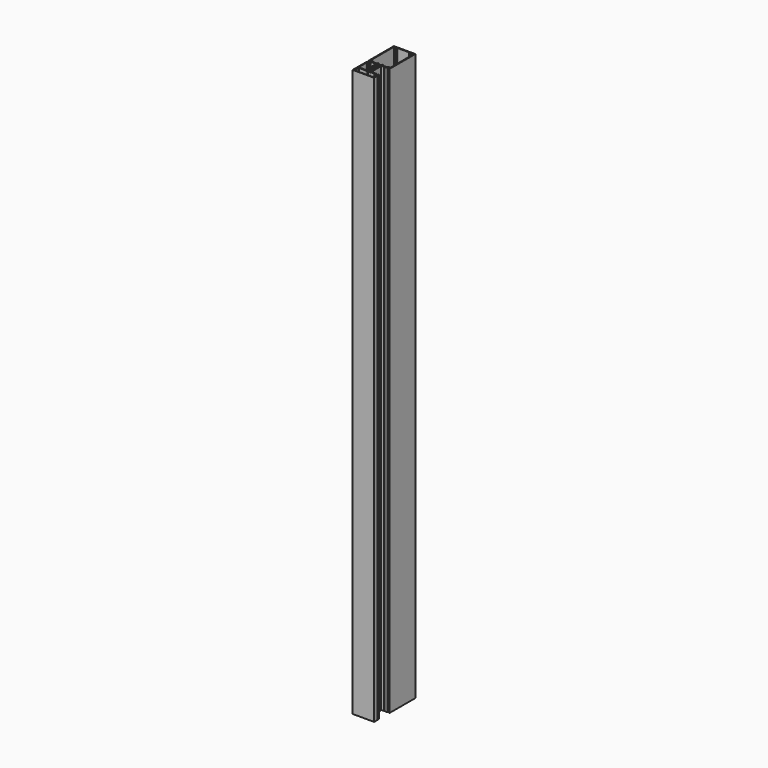
from build123d import *

# Parameters (mm, degrees)
F1_DEPTH = 838.2
F2_DEPTH = 838.2
F3_DEPTH = 838.2


# Not quite as in the source:
# - ends of sketch curves that miss each other by under 0.0002 mm in the source are joined


with BuildPart() as f1:
    # F0 (on Top) → F1 (new body, symmetric)
    with BuildSketch(Plane.XY):
        with BuildLine():
            Line((-36.0498644, -21.2344), (-36.0498644, -50.8))
            Line((-36.0498644, -50.8), (-35.0338644, -50.8))
            Line((-35.0338644, -50.8), (-34.6528644, -51.181))
            Line((-34.6528644, -51.181), (-34.2718644, -50.8))
            Line((-34.2718644, -50.8), (-32.4176644, -50.8))
            Line((-32.4176644, -50.8), (-32.0366644, -51.181))
            Line((-32.0366644, -51.181), (-31.6556644, -50.8))
            Line((-31.6556644, -50.8), (-30.6396644, -50.8))
            Line((-30.6396644, -50.8), (-30.6396644, -39.878))
            Line((-30.6396644, -39.878), (-29.1552122, -34.3379298))
            ThreePointArc((-29.1552122, -34.3379298), (-28.0996644, -33.528), (-27.0441212237, -34.337931039))
            Line((-27.0441212237, -34.337931039), (-25.5596644, -39.878))
            Line((-25.5596644, -39.878), (-25.5596644, -50.8))
            Line((-25.5596644, -50.8), (-24.5436644, -50.8))
            Line((-24.5436644, -50.8), (-24.1626644, -51.181))
            Line((-24.1626644, -51.181), (-23.7816644, -50.8))
            Line((-23.7816644, -50.8), (-21.9274644, -50.8))
            Line((-21.9274644, -50.8), (-21.5464644, -51.181))
            Line((-21.5464644, -51.181), (-21.1654644, -50.8))
            Line((-21.1654644, -50.8), (-20.1494644, -50.8))
            Line((-20.1494644, -50.8), (-20.1494644, -21.2344))
            ThreePointArc((-20.1494644, -21.2344), (-20.2238592776, -21.0547948776), (-20.4034644, -20.9804))
            Line((-20.4034644, -20.9804), (-21.4194644, -20.9804))
            ThreePointArc((-21.4194644, -20.9804), (-21.5990695224, -20.9060051224), (-21.6734644, -20.7264))
            Line((-21.6734644, -20.7264), (-21.6734644, -19.304))
            ThreePointArc((-21.6734644, -19.304), (-21.5990695224, -19.1243948776), (-21.4194644, -19.05))
            Line((-21.4194644, -19.05), (-12.6056644, -19.05))
            Line((-12.6056644, -19.05), (-12.2246644, -18.669))
            Line((-12.2246644, -18.669), (-11.8436644, -19.05))
            Line((-11.8436644, -19.05), (-2.9028644, -19.05))
            ThreePointArc((-2.9028644, -19.05), (-2.5506227914, -18.8142131165), (-2.634359929, -18.3986921218))
            ThreePointArc((-2.634359929, -18.3986921218), (-3.1338033198, -17.6552092218), (-3.3092644, -16.7769032))
            Line((-3.3092644, -16.7769032), (-3.3092644, -16.51))
            ThreePointArc((-3.3092644, -16.51), (-2.9372900121, -15.6119743879), (-2.0392644, -15.24))
            Line((-2.0392644, -15.24), (0.1959356, -15.24))
            ThreePointArc((0.1959356, -15.24), (1.0939612121, -15.6119743879), (1.4659356, -16.51))
            Line((1.4659356, -16.51), (1.4659356, -16.7769032))
            ThreePointArc((1.4659356, -16.7769032), (1.2904710581, -17.6552175402), (0.7910133951, -18.398699839))
            ThreePointArc((0.7910133951, -18.398699839), (0.7072974255, -18.8142214462), (1.0595356, -19.05))
            Line((1.0595356, -19.05), (3.1423356, -19.05))
            ThreePointArc((3.1423356, -19.05), (3.5015458448, -18.9012102448), (3.6503356, -18.542))
            Line((3.6503356, -18.542), (3.6503356, 76.2))
            Line((3.6503356, 76.2), (-59.8496644, 76.2))
            Line((-59.8496644, 76.2), (-59.8496644, -18.542))
            ThreePointArc((-59.8496644, -18.542), (-59.7008746448, -18.9012102448), (-59.3416644, -19.05))
            Line((-59.3416644, -19.05), (-57.2588644, -19.05))
            ThreePointArc((-57.2588644, -19.05), (-56.9066227914, -18.8142131165), (-56.990359929, -18.3986921218))
            ThreePointArc((-56.990359929, -18.3986921218), (-57.4898033198, -17.6552092218), (-57.6652644, -16.7769032))
            Line((-57.6652644, -16.7769032), (-57.6652644, -16.51))
            ThreePointArc((-57.6652644, -16.51), (-57.2932900121, -15.6119743879), (-56.3952644, -15.24))
            Line((-56.3952644, -15.24), (-54.1600644, -15.24))
            ThreePointArc((-54.1600644, -15.24), (-53.2620387879, -15.6119743879), (-52.8900644, -16.51))
            Line((-52.8900644, -16.51), (-52.8900644, -16.7769032))
            ThreePointArc((-52.8900644, -16.7769032), (-53.0655289419, -17.6552175402), (-53.5649866049, -18.398699839))
            ThreePointArc((-53.5649866049, -18.398699839), (-53.6487025745, -18.8142214462), (-53.2964644, -19.05))
            Line((-53.2964644, -19.05), (-50.6956822, -19.05))
            Line((-50.6956822, -19.05), (-44.3556644, -19.05))
            Line((-44.3556644, -19.05), (-43.9746644, -18.669))
            Line((-43.9746644, -18.669), (-43.5936644, -19.05))
            Line((-43.5936644, -19.05), (-34.7798644, -19.05))
            ThreePointArc((-34.7798644, -19.05), (-34.6002592776, -19.1243948776), (-34.5258644, -19.304))
            Line((-34.5258644, -19.304), (-34.5258644, -20.7264))
            ThreePointArc((-34.5258644, -20.7264), (-34.6002592776, -20.9060051224), (-34.7798644, -20.9804))
            Line((-34.7798644, -20.9804), (-35.7958644, -20.9804))
            ThreePointArc((-35.7958644, -20.9804), (-35.9754695224, -21.0547948776), (-36.0498644, -21.2344))
        make_face()
        with BuildLine():
            Line((-33.5098644, -34.9879412), (-33.5098644, -23.2150666))
            ThreePointArc((-33.5098644, -23.2150666), (-32.3971314162, -22.1855160091), (-31.9858644, -20.7264))
            Line((-31.9858644, -20.7264), (-31.9858644, -19.05))
            Line((-31.9858644, -19.05), (-24.2134644, -19.05))
            Line((-24.2134644, -19.05), (-24.2134644, -20.7264))
            ThreePointArc((-24.2134644, -20.7264), (-23.8021973838, -22.1855160091), (-22.6894704645, -23.2150784839))
            Line((-22.6894704645, -23.2150784839), (-22.6894644, -34.9879412))
            ThreePointArc((-22.6894644, -34.9879412), (-23.3519989622, -35.7434215946), (-24.1874975409, -35.1851700405))
            Line((-24.1874975409, -35.1851700405), (-24.5906798, -33.6805524))
            ThreePointArc((-24.5906798, -33.6805524), (-28.099667687, -30.988), (-31.608665629, -33.6805547502))
            Line((-31.608665629, -33.6805547502), (-32.0118232, -35.1851722))
            ThreePointArc((-32.0118232, -35.1851722), (-32.8473298378, -35.7434215946), (-33.5098644, -34.9879412))
        make_face(mode=Mode.SUBTRACT)
        with BuildLine():
            Line((-34.0178644, -16.51), (-34.0178644, -13.208))
            ThreePointArc((-34.0178644, -13.208), (-34.1666541552, -12.8487897552), (-34.5258644, -12.7))
            Line((-34.5258644, -12.7), (-35.5418644, -12.7))
            ThreePointArc((-35.5418644, -12.7), (-35.9010746448, -12.8487897552), (-36.0498644, -13.208))
            Line((-36.0498644, -13.208), (-36.0498644, -15.875))
            Line((-36.0498644, -15.875), (-50.8326644, -15.875))
            Line((-50.8326644, -15.875), (-50.8326644, -13.208))
            ThreePointArc((-50.8326644, -13.208), (-50.9814541552, -12.8487897552), (-51.3406644, -12.7))
            Line((-51.3406644, -12.7), (-56.5476644, -12.7))
            ThreePointArc((-56.5476644, -12.7), (-57.0864797673, -12.4768153673), (-57.3096644, -11.938))
            Line((-57.3096644, -11.938), (-57.3096644, 73.66))
            Line((-57.3096644, 73.66), (-53.2456644, 73.66))
            ThreePointArc((-53.2456644, 73.66), (-52.1680336655, 73.2136307345), (-51.7216644, 72.136))
            Line((-51.7216644, 72.136), (-51.7216644, 70.612))
            Line((-51.7216644, 70.612), (-45.7526644, 70.612))
            Line((-45.7526644, 70.612), (-45.7526644, 72.136))
            ThreePointArc((-45.7526644, 72.136), (-45.3062951345, 73.2136307345), (-44.2286644, 73.66))
            Line((-44.2286644, 73.66), (-11.9706644, 73.66))
            ThreePointArc((-11.9706644, 73.66), (-10.8930336655, 73.2136307345), (-10.4466644, 72.136))
            Line((-10.4466644, 72.136), (-10.4466644, 70.612))
            Line((-10.4466644, 70.612), (-4.4776644, 70.612))
            Line((-4.4776644, 70.612), (-4.4776644, 72.136))
            ThreePointArc((-4.4776644, 72.136), (-4.0312951345, 73.2136307345), (-2.9536644, 73.66))
            Line((-2.9536644, 73.66), (1.1103356, 73.66))
            Line((1.1103356, 73.66), (1.1103356, -11.938))
            ThreePointArc((1.1103356, -11.938), (0.8871509673, -12.4768153673), (0.3483356, -12.7))
            Line((0.3483356, -12.7), (-4.8586644, -12.7))
            ThreePointArc((-4.8586644, -12.7), (-5.2178746448, -12.8487897552), (-5.3666644, -13.208))
            Line((-5.3666644, -13.208), (-5.3666644, -15.875))
            Line((-5.3666644, -15.875), (-20.1494644, -15.875))
            Line((-20.1494644, -15.875), (-20.1494644, -13.208))
            ThreePointArc((-20.1494644, -13.208), (-20.2982541552, -12.8487897552), (-20.6574644, -12.7))
            Line((-20.6574644, -12.7), (-21.6734644, -12.7))
            ThreePointArc((-21.6734644, -12.7), (-22.0326746448, -12.8487897552), (-22.1814644, -13.208))
            Line((-22.1814644, -13.208), (-22.1814644, -16.51))
            Line((-22.1814644, -16.51), (-34.0178644, -16.51))
        make_face(mode=Mode.SUBTRACT)
    extrude(amount=F1_DEPTH, both=True)


with BuildPart() as f2:
    # F0 (on Top) → F2 (new body, symmetric)
    with BuildSketch(Plane.XY):
        with BuildLine():
            ThreePointArc((-58.0716644, -63.1444), (-57.1736387836, -63.5163743922), (-56.8016644, -64.4144000122))
            ThreePointArc((-56.8016644, -64.4144000122), (-57.0399094476, -65.1549279996), (-57.6652576455, -65.6176179976))
            Line((-57.6652576455, -65.6176179976), (-54.987063, -70.2564))
            ThreePointArc((-54.987063, -70.2564), (-53.5991814224, -70.6282817077), (-53.2272998923, -69.2403998224))
            Line((-53.2272998923, -69.2403998224), (-54.7696644, -66.5689296))
            Line((-54.7696644, -66.5689296), (-54.7696644, -59.69))
            Line((-54.7696644, -59.69), (-36.3546644, -59.69))
            Line((-36.3546644, -59.69), (-35.7196644, -60.325))
            Line((-35.7196644, -60.325), (-34.4496644, -60.325))
            Line((-34.4496644, -60.325), (-31.4778644, -60.325))
            Line((-31.4778644, -60.325), (-31.4778644, -57.15))
            Line((-31.4778644, -57.15), (-33.0526644, -57.15))
            Line((-33.0526644, -57.15), (-33.4336644, -56.769))
            Line((-33.4336644, -56.769), (-33.8146644, -57.15))
            Line((-33.8146644, -57.15), (-34.4623644, -57.15))
            Line((-34.4623644, -57.15), (-36.0498644, -57.15))
            Line((-36.0498644, -57.15), (-55.7856644, -57.15))
            ThreePointArc((-55.7856644, -57.15), (-56.8632951345, -56.7036307345), (-57.3096644, -55.626))
            Line((-57.3096644, -55.626), (-57.3096644, -29.464))
            ThreePointArc((-57.3096644, -29.464), (-56.8632951345, -28.3863692655), (-55.7856644, -27.94))
            Line((-55.7856644, -27.94), (-50.4516644, -27.94))
            ThreePointArc((-50.4516644, -27.94), (-49.9128490327, -27.7168153673), (-49.6896644, -27.178))
            Line((-49.6896644, -27.178), (-49.6896644, -26.162))
            ThreePointArc((-49.6896644, -26.162), (-49.9128490327, -25.6231846327), (-50.4516644, -25.4))
            Line((-50.4516644, -25.4), (-59.8496644, -25.4))
            Line((-59.8496644, -25.4), (-59.8496644, -62.3824))
            ThreePointArc((-59.8496644, -62.3824), (-59.6264797673, -62.9212153673), (-59.0876644, -63.1444))
            Line((-59.0876644, -63.1444), (-58.0716644, -63.1444))
        make_face()
    extrude(amount=F2_DEPTH, both=True)


with BuildPart() as f2b:
    # F0 (on Top) → F2, piece 2 (new body, symmetric)
    with BuildSketch(Plane.XY):
        with BuildLine():
            ThreePointArc((1.4659288455, -65.6176179976), (0.840580644, -65.1549279947), (0.6023356, -64.4144))
            ThreePointArc((0.6023356, -64.4144), (0.9743099879, -63.5163743879), (1.8723356, -63.1444))
            Line((1.8723356, -63.1444), (2.8883356, -63.1444))
            ThreePointArc((2.8883356, -63.1444), (3.4271509673, -62.9212153673), (3.6503356, -62.3824))
            Line((3.6503356, -62.3824), (3.6503356, -57.658))
            ThreePointArc((3.6503356, -57.658), (3.5015458448, -57.2987897552), (3.1423356, -57.15))
            Line((3.1423356, -57.15), (1.0595356, -57.15))
            ThreePointArc((1.0595356, -57.15), (0.7073008372, -57.3857702789), (0.7910056453, -57.8012825622))
            ThreePointArc((0.7910056453, -57.8012825622), (1.2904710581, -58.5447570598), (1.4659356, -59.4230714))
            Line((1.4659356, -59.4230714), (1.4659356, -59.69))
            ThreePointArc((1.4659356, -59.69), (1.0939612121, -60.5880256121), (0.1959356, -60.96))
            Line((0.1959356, -60.96), (-2.0392644, -60.96))
            ThreePointArc((-2.0392644, -60.96), (-2.9372900121, -60.5880256121), (-3.3092644, -59.69))
            Line((-3.3092644, -59.69), (-3.3092644, -59.4230714))
            ThreePointArc((-3.3092644, -59.4230714), (-3.1338033198, -58.5447653782), (-2.6343549792, -57.8012874608))
            ThreePointArc((-2.6343549792, -57.8012874608), (-2.5506262029, -57.3857786086), (-2.9028644, -57.15))
            Line((-2.9028644, -57.15), (-20.1494644, -57.15))
            Line((-20.1494644, -57.15), (-21.7369644, -57.15))
            Line((-21.7369644, -57.15), (-22.3846644, -57.15))
            Line((-22.3846644, -57.15), (-22.7656644, -56.769))
            Line((-22.7656644, -56.769), (-23.1466644, -57.15))
            Line((-23.1466644, -57.15), (-24.7214644, -57.15))
            Line((-24.7214644, -57.15), (-24.7214644, -60.325))
            Line((-24.7214644, -60.325), (-21.7496644, -60.325))
            Line((-21.7496644, -60.325), (-20.4796644, -60.325))
            Line((-20.4796644, -60.325), (-19.8446644, -59.69))
            Line((-19.8446644, -59.69), (-5.8492644, -59.69))
            Line((-5.8492644, -59.69), (-5.8492644, -61.6204))
            ThreePointArc((-5.8492644, -61.6204), (-5.4028951345, -62.6980307345), (-4.3252644, -63.1444))
            Line((-4.3252644, -63.1444), (-1.4296644, -63.1444))
            Line((-1.4296644, -63.1444), (-1.4296644, -66.5689296))
            Line((-1.4296644, -66.5689296), (-2.9720286, -69.2404))
            ThreePointArc((-2.9720286, -69.2404), (-2.6001473776, -70.6282817077), (-1.2122654923, -70.2564001776))
            Line((-1.2122654923, -70.2564001776), (1.4659288455, -65.6176179976))
        make_face()
    extrude(amount=F2_DEPTH, both=True)


with BuildPart() as f2c:
    # F0 (on Top) → F2, piece 3 (new body, symmetric)
    with BuildSketch(Plane.XY):
        with BuildLine():
            Line((-59.8496644, -76.2), (3.6503356, -76.2))
            Line((3.6503356, -76.2), (3.6503356, -64.9224))
            ThreePointArc((3.6503356, -64.9224), (3.2039663345, -63.8447692655), (2.1263356, -63.3984))
            Line((2.1263356, -63.3984), (1.6183356, -63.3984))
            ThreePointArc((1.6183356, -63.3984), (0.8999151103, -63.6959795103), (0.6023356, -64.4144))
            ThreePointArc((0.6023356, -64.4144), (0.8999151103, -65.1328204897), (1.6183356, -65.4304))
            Line((1.6183356, -65.4304), (2.3803356, -65.4304))
            Line((2.3803356, -65.4304), (2.3803356, -74.676))
            Line((2.3803356, -74.676), (-58.5796644, -74.676))
            Line((-58.5796644, -74.676), (-58.5796644, -65.4304))
            Line((-58.5796644, -65.4304), (-57.8176644, -65.4304))
            ThreePointArc((-57.8176644, -65.4304), (-57.0992439146, -65.132820494), (-56.8016644, -64.4144000122))
            ThreePointArc((-56.8016644, -64.4144000122), (-57.099243906, -63.6959795146), (-57.8176644, -63.3984))
            Line((-57.8176644, -63.3984), (-58.3256644, -63.3984))
            ThreePointArc((-58.3256644, -63.3984), (-59.4032951345, -63.8447692655), (-59.8496644, -64.9224))
            Line((-59.8496644, -64.9224), (-59.8496644, -76.2))
        make_face()
    extrude(amount=F2_DEPTH, both=True)


with BuildPart() as f3:
    # F0 (on Top) → F3 (new body, symmetric)
    with BuildSketch(Plane.XY):
        Polygon((-31.4778644, -57.15), (-31.4778644, -60.325), (-28.4806644, -60.325), (-28.0996644, -59.944), (-27.7186644, -60.325), (-24.7214644, -60.325), (-24.7214644, -57.15), align=None)
    extrude(amount=F3_DEPTH, both=True)


solid = Compound([f1.part, f2.part, f2b.part, f2c.part, f3.part])
